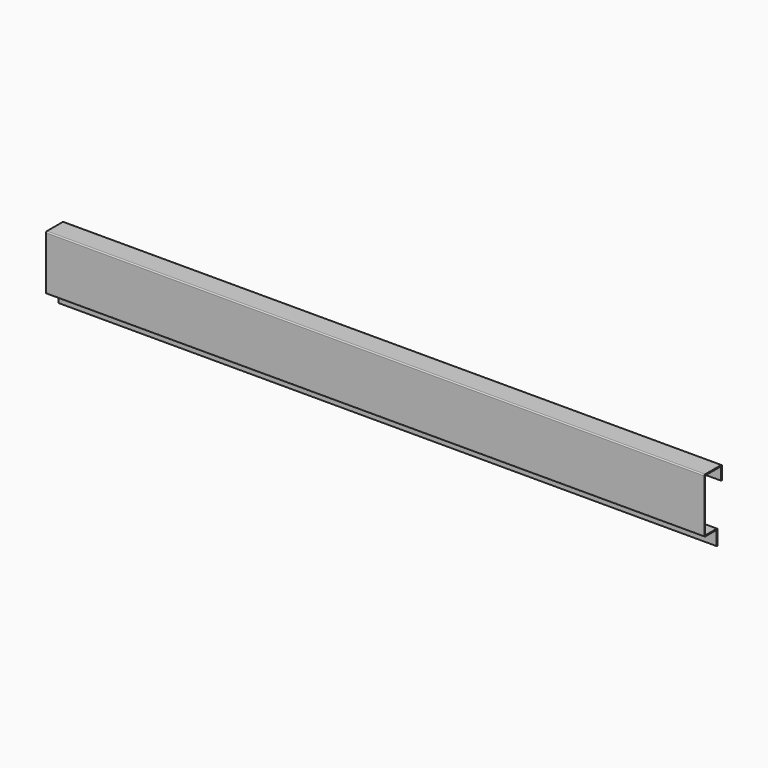
from build123d import *

# Parameters (mm, degrees)
F1_DEPTH = 1200
F2_R     = 2


# Not quite as in the source:
# - a feature names something its author has since deleted; it is built from what else it names


with BuildPart() as f1:
    # F0 (on Right) → F1 (new body)
    with BuildSketch(Plane.YZ):
        Polygon((-19.8378913403, 177.8021101952), (-19.8378913403, 154.8021101952), (-17.8378913403, 154.8021101952), (-17.8378913403, 179.8021101952), (-57.8378913403, 179.8021101952), (-57.8378913403, 79.8021101952), (-29.8378913403, 79.8021101952), (-29.8378913403, 53.8021101952), (-27.8378913403, 53.8021101952), (-27.8378913403, 81.8021101952), (-55.8378913403, 81.8021101952), (-55.8378913403, 177.8021101952), align=None)
    extrude(amount=F1_DEPTH)

    # F2
    f2_edges = [f1.edges().sort_by_distance(p)[0] for p in [
        (600, -57.837891, 179.80211),
        (600, -17.837891, 179.80211),
        (600, -57.837891, 79.80211),
        (600, -27.837891, 81.80211),
        (600, -55.837891, 81.80211),
        (600, -29.837891, 79.80211),
        (600, -19.837891, 177.80211),
        (600, -55.837891, 177.80211),
    ]]
    fillet(f2_edges, radius=F2_R)


solid = f1.part
